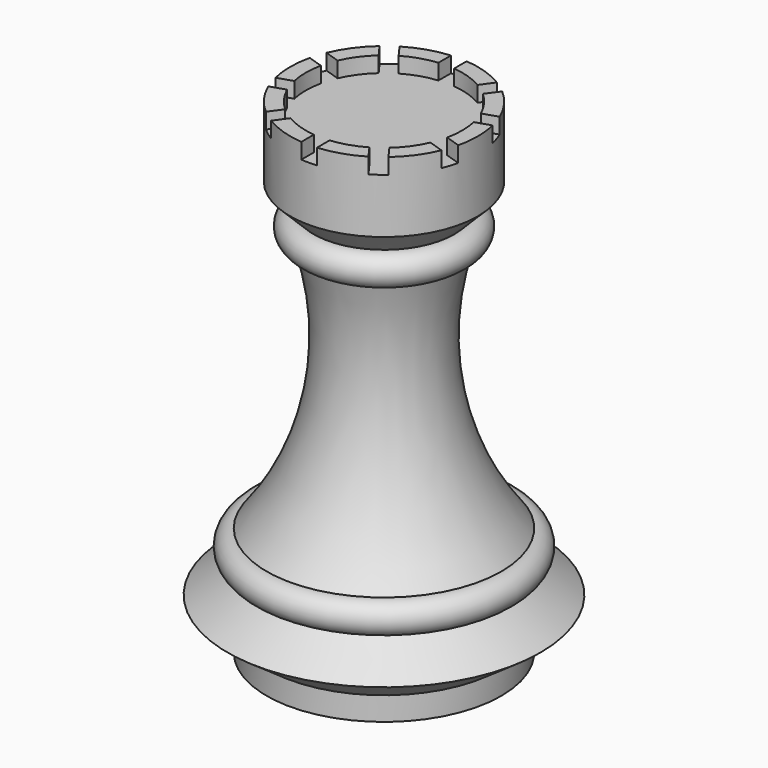
from build123d import *

# Parameters (mm, degrees)
F2_W            = 2.54
F2_H            = 2.54
F3_DEPTH        = 25.4
F3_DEPTH_BACK   = 25.4
F3_COPIES_COUNT = 5
F3_COPIES_ANGLE = 144


# Not quite as in the source:
# - a pattern or mirror of a feature is missing from the dataset's text; its kind, count and spacing are read off the source's solid


with BuildPart() as f1:
    # F0 (on Front) → F1 (revolve)
    with BuildSketch(Plane.XZ):
        with BuildLine():
            Line((0, 76.2), (0, 0))
            Line((0, 0), (19.05, 0))
            Line((19.05, 0), (19.05, 3.81))
            Line((19.05, 3.81), (25.4, 8.255))
            Line((25.4, 8.255), (19.05, 12.7))
            ThreePointArc((19.05, 12.7), (21.59, 15.24), (19.05, 17.78))
            ThreePointArc((19.05, 17.78), (10.2268710231, 37.1600383168), (11.43, 58.42))
            ThreePointArc((11.43, 58.42), (13.97, 60.96), (11.43, 63.5))
            Line((11.43, 63.5), (15.24, 67.31))
            Line((15.24, 67.31), (15.24, 78.74))
            Line((15.24, 78.74), (12.7, 78.74))
            Line((12.7, 78.74), (12.7, 76.2))
            Line((12.7, 76.2), (0, 76.2))
        make_face()
    revolve(axis=Axis((0, 0, 38.1), (0, 0, 1)))

    # F2 (on Front) → F3 (cut, two sides)
    with BuildSketch(Plane.XZ) as f3_sk:
        with Locations((0, 77.47)):
            Rectangle(F2_W, F2_H)
    f3 = extrude(amount=-F3_DEPTH, mode=Mode.SUBTRACT) + extrude(f3_sk.sketch, amount=F3_DEPTH_BACK, mode=Mode.SUBTRACT)

    # F3_copies: F3 ×5 about axis
    f3_copies_axis = Axis((0, 0, 0), (0, 0, 1))
    for i in range(1, F3_COPIES_COUNT):
        add(f3.rotate(f3_copies_axis, i * F3_COPIES_ANGLE / (F3_COPIES_COUNT - 1)), mode=Mode.SUBTRACT)


solid = f1.part
